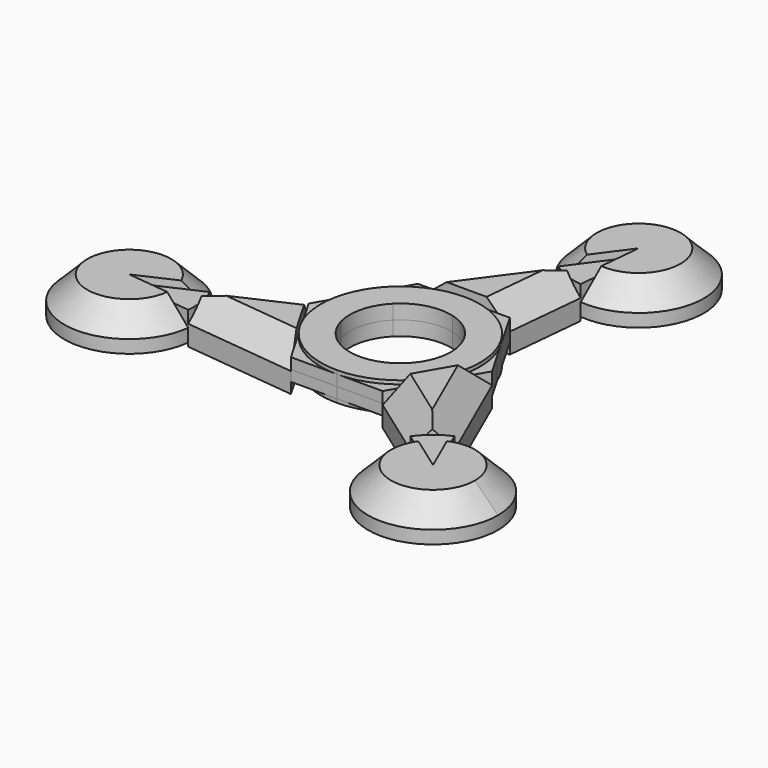
from build123d import *

# Parameters (mm, degrees)
F1_DEPTH      = 3.175
F1_DEPTH_BACK = 3.175
F2_DEPTH      = 2.38125
F2_DEPTH_BACK = 2.38125
F3_DEPTH      = 4.7625
F3_DEPTH_BACK = 4.7625
F4_DEPTH      = 3.96875
F4_DEPTH_BACK = 3.96875
F5_DEPTH      = 2.38125
F5_DEPTH_BACK = 2.38125
F6_T1_DEPTH   = 51.0658567028
F6_T3_DEPTH   = 43.5956947451
F6_2_T1_DEPTH = 43.5956947451
F6_2_T3_DEPTH = 51.0658567028
F6_3_T1_DEPTH = 43.5956947451
F6_3_T3_DEPTH = 51.0658567028
F6_4_T2_ANGLE = 359.64
F6_5_T2_ANGLE = 359.64
F6_6_T2_ANGLE = 268.0514708104
F6_6_T4_ANGLE = 166.1085533485


# Not quite as in the source:
# - a fillet or chamfer that OpenCascade refuses, or shapes differently, is made with other operations: its cross-section is extruded or revolved along the edge and cut away or added
# - a length typed as a fraction of an inch, garbled in the dataset ("3 / 203.2 mm" for 3/8 in), is restored


with BuildPart() as f1:
    # F0 (on Top) → F1 (new body, two sides)
    with BuildSketch(Plane.XY) as f1_sk:
        with BuildLine():
            Line((-4.5196275751, -16.8674797416), (-2.8761266387, -10.7338507446))
            ThreePointArc((-2.8761266387, -10.7338507446), (-7.8577241059, -7.8577241059), (-10.7338507446, -2.8761266387))
            Line((-10.7338507446, -2.8761266387), (-16.8674797416, -4.5196275751))
            ThreePointArc((-16.8674797416, -4.5196275751), (-16.1332463557, -6.6826093913), (-15.1229686637, -8.7312499131))
            ThreePointArc((-15.1229686637, -8.7312499131), (-10.6304964939, -13.8539326743), (-4.5196275751, -16.8674797416))
        make_face()
        with BuildLine():
            ThreePointArc((-7.8577241059, 7.8577241059), (-2.8761266387, 10.7338507446), (2.8761266387, 10.7338507446))
            Line((2.8761266387, 10.7338507446), (4.5196275751, 16.8674797416))
            ThreePointArc((4.5196275751, 16.8674797416), (2.2793136316, 17.3131058917), (0, 17.4625))
            ThreePointArc((0, 17.4625), (-6.6826094377, 16.1332463365), (-12.3478521665, 12.3478521665))
            Line((-12.3478521665, 12.3478521665), (-7.8577241059, 7.8577241059))
        make_face()
        with BuildLine():
            ThreePointArc((-10.7338507446, -2.8761266387), (-10.7338507446, 2.8761266387), (-7.8577241059, 7.8577241059))
            Line((-7.8577241059, 7.8577241059), (-12.3478521665, 12.3478521665))
            ThreePointArc((-12.3478521665, 12.3478521665), (-13.8539326905, 10.6304964728), (-15.12296859, 8.7312500408))
            ThreePointArc((-15.12296859, 8.7312500408), (-17.3131058887, 2.279313655), (-16.8674797416, -4.5196275751))
            Line((-16.8674797416, -4.5196275751), (-10.7338507446, -2.8761266387))
        make_face()
        with BuildLine():
            ThreePointArc((2.8761266387, 10.7338507446), (7.8577241059, 7.8577241059), (10.7338507446, 2.8761266387))
            Line((10.7338507446, 2.8761266387), (16.8674797416, 4.5196275751))
            ThreePointArc((16.8674797416, 4.5196275751), (16.1332463692, 6.6826093587), (15.122968699, 8.731249852))
            ThreePointArc((15.122968699, 8.731249852), (10.6304965218, 13.8539326528), (4.5196275751, 16.8674797416))
            Line((4.5196275751, 16.8674797416), (2.8761266387, 10.7338507446))
        make_face()
        with BuildLine():
            ThreePointArc((10.7338507446, 2.8761266387), (11.017431022, 1.450472311), (11.1125, 0))
            ThreePointArc((11.1125, 0), (10.266611305, -4.2525696422), (7.8577241059, -7.8577241059))
            Line((7.8577241059, -7.8577241059), (12.3478521665, -12.3478521665))
            ThreePointArc((12.3478521665, -12.3478521665), (13.853932765, -10.6304963756), (15.1229687125, -8.7312498287))
            ThreePointArc((15.1229687125, -8.7312498287), (16.8674797672, -4.5196274796), (17.4625, 0))
            ThreePointArc((17.4625, 0), (17.3131058917, 2.2793136316), (16.8674797416, 4.5196275751))
            Line((16.8674797416, 4.5196275751), (10.7338507446, 2.8761266387))
        make_face()
        with BuildLine():
            Line((12.3478521665, -12.3478521665), (7.8577241059, -7.8577241059))
            ThreePointArc((7.8577241059, -7.8577241059), (2.8761266387, -10.7338507446), (-2.8761266387, -10.7338507446))
            Line((-2.8761266387, -10.7338507446), (-4.5196275751, -16.8674797416))
            ThreePointArc((-4.5196275751, -16.8674797416), (-2.2793136142, -17.313105894), (3.53e-08, -17.4625))
            ThreePointArc((3.53e-08, -17.4625), (6.682609454, -16.1332463297), (12.3478521665, -12.3478521665))
        make_face()
    extrude(amount=-F1_DEPTH)
    extrude(f1_sk.sketch, amount=F1_DEPTH_BACK)

    # F0 (on Top) → F2 (join, two sides)
    with BuildSketch(Plane.XY) as f2_sk:
        with BuildLine():
            Line((4.6790627728, 17.4625), (4.5196275751, 16.8674797416))
            ThreePointArc((4.5196275751, 16.8674797416), (10.6304965218, 13.8539326528), (15.122968699, 8.731249852))
            Line((15.122968699, 8.731249852), (10.0819790757, 17.4625))
            Line((10.0819790757, 17.4625), (4.6790627728, 17.4625))
        make_face()
        with BuildLine():
            Line((17.4625, 4.6790627728), (16.8674797416, 4.5196275751))
            ThreePointArc((16.8674797416, 4.5196275751), (17.3131058917, 2.2793136316), (17.4625, 0))
            ThreePointArc((17.4625, 0), (16.8674797672, -4.5196274796), (15.1229687125, -8.7312498287))
            Line((15.1229687125, -8.7312498287), (20.1639581514, 0))
            Line((20.1639581514, 0), (17.4625, 4.6790627728))
        make_face()
        with BuildLine():
            Line((12.7834372272, -12.7834372272), (12.3478521665, -12.3478521665))
            ThreePointArc((12.3478521665, -12.3478521665), (6.682609454, -16.1332463297), (3.53e-08, -17.4625))
            Line((3.53e-08, -17.4625), (10.0819790757, -17.4625))
            Line((10.0819790757, -17.4625), (12.7834372272, -12.7834372272))
        make_face()
        with BuildLine():
            Line((-4.6790627728, -17.4625), (-4.5196275751, -16.8674797416))
            ThreePointArc((-4.5196275751, -16.8674797416), (-10.6304964939, -13.8539326743), (-15.1229686637, -8.7312499131))
            Line((-15.1229686637, -8.7312499131), (-10.0819790757, -17.4625))
            Line((-10.0819790757, -17.4625), (-4.6790627728, -17.4625))
        make_face()
        with BuildLine():
            Line((-17.4625, -4.6790627728), (-16.8674797416, -4.5196275751))
            ThreePointArc((-16.8674797416, -4.5196275751), (-17.3131058887, 2.279313655), (-15.12296859, 8.7312500408))
            Line((-15.12296859, 8.7312500408), (-20.1639581514, 0))
            Line((-20.1639581514, 0), (-17.4625, -4.6790627728))
        make_face()
        with BuildLine():
            Line((-12.7834372272, 12.7834372272), (-12.3478521665, 12.3478521665))
            ThreePointArc((-12.3478521665, 12.3478521665), (-6.6826094377, 16.1332463365), (0, 17.4625))
            Line((0, 17.4625), (-10.0819790757, 17.4625))
            Line((-10.0819790757, 17.4625), (-12.7834372272, 12.7834372272))
        make_face()
        with BuildLine():
            ThreePointArc((-15.12296859, 8.7312500408), (-13.8539326905, 10.6304964728), (-12.3478521665, 12.3478521665))
            Line((-12.3478521665, 12.3478521665), (-12.7834372272, 12.7834372272))
            Line((-12.7834372272, 12.7834372272), (-15.12296859, 8.7312500408))
        make_face()
        with BuildLine():
            ThreePointArc((-15.1229686637, -8.7312499131), (-16.1332463557, -6.6826093913), (-16.8674797416, -4.5196275751))
            Line((-16.8674797416, -4.5196275751), (-17.4625, -4.6790627728))
            Line((-17.4625, -4.6790627728), (-15.1229686637, -8.7312499131))
        make_face()
        with BuildLine():
            ThreePointArc((3.53e-08, -17.4625), (-2.2793136142, -17.313105894), (-4.5196275751, -16.8674797416))
            Line((-4.5196275751, -16.8674797416), (-4.6790627728, -17.4625))
            Line((-4.6790627728, -17.4625), (3.53e-08, -17.4625))
        make_face()
        with BuildLine():
            ThreePointArc((15.1229687125, -8.7312498287), (13.853932765, -10.6304963756), (12.3478521665, -12.3478521665))
            Line((12.3478521665, -12.3478521665), (12.7834372272, -12.7834372272))
            Line((12.7834372272, -12.7834372272), (15.1229687125, -8.7312498287))
        make_face()
        with BuildLine():
            ThreePointArc((15.122968699, 8.731249852), (16.1332463692, 6.6826093587), (16.8674797416, 4.5196275751))
            Line((16.8674797416, 4.5196275751), (17.4625, 4.6790627728))
            Line((17.4625, 4.6790627728), (15.122968699, 8.731249852))
        make_face()
        with BuildLine():
            ThreePointArc((0, 17.4625), (2.2793136316, 17.3131058917), (4.5196275751, 16.8674797416))
            Line((4.5196275751, 16.8674797416), (4.6790627728, 17.4625))
            Line((4.6790627728, 17.4625), (0, 17.4625))
        make_face()
    extrude(amount=F2_DEPTH)
    extrude(f2_sk.sketch, amount=-F2_DEPTH_BACK)


with BuildPart() as f3:
    # F0 (on Top) → F3 (new body, two sides)
    with BuildSketch(Plane.XY) as f3_sk:
        with BuildLine():
            Line((25.8182363481, -25.8182363481), (12.7834372272, -12.7834372272))
            Line((12.7834372272, -12.7834372272), (10.0819790757, -17.4625))
            Line((10.0819790757, -17.4625), (24.2952466492, -27.6159690372))
            ThreePointArc((24.2952466492, -27.6159690372), (25.0196206528, -26.6856549328), (25.8182363481, -25.8182363481))
        make_face()
        with BuildLine():
            Line((20.1639581514, 0), (15.1229687125, -8.7312498287))
            Line((15.1229687125, -8.7312498287), (12.7834372272, -12.7834372272))
            Line((12.7834372272, -12.7834372272), (25.8182363481, -25.8182363481))
            ThreePointArc((25.8182363481, -25.8182363481), (27.8608858867, -24.1241256529), (30.1816043452, -22.8369993881))
            Line((30.1816043452, -22.8369993881), (20.1639581514, 0))
        make_face()
    extrude(amount=F3_DEPTH)
    extrude(f3_sk.sketch, amount=-F3_DEPTH_BACK)

    # F6: chamfer of 5.08 on 2 edges, made by hand

    # F6_s2 → F6_t1 (cut)
    with BuildSketch(Plane(origin=(18.5194987555, -42.2184786293, 0), x_dir=(0, 0, 1), z_dir=(-0.4017091961, 0.9157672858, 0))):
        Polygon((-0.3175, 18.4654932278), (4.7625, 13.3854932278), (4.7625, 18.4654932278), align=None)
    extrude(amount=F6_T1_DEPTH, mode=Mode.SUBTRACT)

    # F6_s4 → F6_t3 (cut)
    with BuildSketch(Plane(origin=(4.3046564772, -3.0750983918, 0), x_dir=(0, 0, 1), z_dir=(0.8137027356, -0.5812812211, 0))):
        Polygon((-0.3175, 8.348818912), (4.7625, 3.268818912), (4.7625, 8.348818912), align=None)
    extrude(amount=F6_T3_DEPTH, mode=Mode.SUBTRACT)


with BuildPart() as f3b:
    # F0 (on Top) → F3, piece 2 (new body, two sides)
    with BuildSketch(Plane.XY) as f3_2_sk:
        with BuildLine():
            Line((9.4501303843, 35.2683667324), (4.6790627728, 17.4625))
            Line((4.6790627728, 17.4625), (10.0819790757, 17.4625))
            Line((10.0819790757, 17.4625), (11.7685074117, 34.848285308))
            ThreePointArc((11.7685074117, 34.848285308), (10.600644762, 35.0104545447), (9.4501303843, 35.2683667324))
        make_face()
        with BuildLine():
            Line((-10.0819790757, 17.4625), (0, 17.4625))
            Line((0, 17.4625), (4.6790627728, 17.4625))
            Line((4.6790627728, 17.4625), (9.4501303843, 35.2683667324))
            ThreePointArc((9.4501303843, 35.2683667324), (6.9616627161, 36.1902977763), (4.6866194437, 37.556535784))
            Line((4.6866194437, 37.556535784), (-10.0819790757, 17.4625))
        make_face()
    extrude(amount=F3_DEPTH)
    extrude(f3_2_sk.sketch, amount=-F3_DEPTH_BACK)

    # F6#2: chamfer of 5.08 on 2 edges, made by hand

    # F6_2_s2 → F6_2_t1 (cut)
    with BuildSketch(Plane(origin=(0.5107850878, 5.2654910597, 0), x_dir=(0, 0, 1), z_dir=(0.0965529364, 0.9953278507, 0))):
        Polygon((4.7625, 3.268818912), (-0.3175, 8.348818912), (4.7625, 8.348818912), align=None)
    extrude(amount=F6_2_T1_DEPTH, mode=Mode.SUBTRACT)

    # F6_2_s4 → F6_2_t3 (cut)
    with BuildSketch(Plane(origin=(27.3025256244, 37.1475957023, 0), x_dir=(0, 0, 1), z_dir=(-0.5922231354, -0.8057740117, 0))):
        Polygon((-0.3175, 18.4654932278), (4.7625, 13.3854932278), (4.7625, 18.4654932278), align=None)
    extrude(amount=F6_2_T3_DEPTH, mode=Mode.SUBTRACT)


with BuildPart() as f3c:
    # F0 (on Top) → F3, piece 3 (new body, two sides)
    with BuildSketch(Plane.XY) as f3_3_sk:
        with BuildLine():
            Line((-10.0819790757, -17.4625), (-15.1229686637, -8.7312499131))
            Line((-15.1229686637, -8.7312499131), (-17.4625, -4.6790627728))
            Line((-17.4625, -4.6790627728), (-35.2683667324, -9.4501303843))
            ThreePointArc((-35.2683667324, -9.4501303843), (-34.9037635186, -11.2831145199), (-34.7815319755, -13.1480074912))
            ThreePointArc((-34.7815319755, -13.1480074912), (-34.8032213919, -13.9349666021), (-34.8682237889, -14.7195363959))
            Line((-34.8682237889, -14.7195363959), (-10.0819790757, -17.4625))
        make_face()
        with BuildLine():
            Line((-35.2683667324, -9.4501303843), (-17.4625, -4.6790627728))
            Line((-17.4625, -4.6790627728), (-20.1639581514, 0))
            Line((-20.1639581514, 0), (-36.0637540609, -7.2323162708))
            ThreePointArc((-36.0637540609, -7.2323162708), (-35.6202654148, -8.324799612), (-35.2683667324, -9.4501303843))
        make_face()
    extrude(amount=F3_DEPTH)
    extrude(f3_3_sk.sketch, amount=-F3_DEPTH_BACK)

    # F6#3: chamfer of 5.08 on 2 edges, made by hand

    # F6_3_s2 → F6_3_t1 (cut)
    with BuildSketch(Plane(origin=(-4.815441565, -2.1903926679, 0), x_dir=(0, 0, 1), z_dir=(-0.9102556721, -0.4140466296, 0))):
        Polygon((-0.3175, 8.348818912), (4.7625, 3.268818912), (4.7625, 8.348818912), align=None)
    extrude(amount=F6_3_T1_DEPTH, mode=Mode.SUBTRACT)

    # F6_3_s4 → F6_3_t3 (cut)
    with BuildSketch(Plane(origin=(-45.8220243799, 5.070882927, 0), x_dir=(0, 0, 1), z_dir=(0.9939323315, -0.1099932742, 0))):
        Polygon((-0.3175, 18.4654932278), (4.7625, 13.3854932278), (4.7625, 18.4654932278), align=None)
    extrude(amount=F6_3_T3_DEPTH, mode=Mode.SUBTRACT)


with BuildPart() as f4:
    # F0 (on Top) → F4 (new body, two sides)
    with BuildSketch(Plane.XY) as f4_sk:
        with BuildLine():
            Line((13.1480074912, 49.0690319755), (11.7685074117, 34.848285308))
            ThreePointArc((11.7685074117, 34.848285308), (22.7506906804, 38.4897535588), (27.4355074912, 49.0690319755))
            ThreePointArc((27.4355074912, 49.0690319755), (6.6966287811, 61.8170659019), (4.6866194437, 37.556535784))
            Line((4.6866194437, 37.556535784), (13.1480074912, 49.0690319755))
        make_face()
    extrude(amount=F4_DEPTH)
    extrude(f4_sk.sketch, amount=-F4_DEPTH_BACK)

    # F6#4: chamfer of 5.08 on 1 edges, made by hand

    # F6_4_s1 → F6_4_t2 (revolve, cut)
    with BuildSketch(Plane(origin=(-5.042448021, 1.9465092507, 0), x_dir=(0, 0, 1), z_dir=(0.9329044068, -0.3601241005, 0))):
        Polygon((3.96875, -41.3041305388), (-1.11125, -36.2241305388), (3.96875, -36.2241305388), align=None)
    revolve(axis=Axis((13.1480074912, 49.0690319755, 3.96875), (0, 0, -1)), revolution_arc=F6_4_T2_ANGLE, mode=Mode.SUBTRACT)


with BuildPart() as f4b:
    # F0 (on Top) → F4, piece 2 (new body, two sides)
    with BuildSketch(Plane.XY) as f4_2_sk:
        with BuildLine():
            ThreePointArc((-36.0637540609, -7.2323162708), (-63.1778021748, -15.4008411988), (-34.8682237889, -14.7195363959))
            Line((-34.8682237889, -14.7195363959), (-49.0690319755, -13.1480074912))
            Line((-49.0690319755, -13.1480074912), (-36.0637540609, -7.2323162708))
        make_face()
    extrude(amount=F4_DEPTH)
    extrude(f4_2_sk.sketch, amount=-F4_DEPTH_BACK)

    # F6#5: chamfer of 5.08 on 1 edges, made by hand

    # F6_5_s1 → F6_5_t2 (revolve, cut)
    with BuildSketch(Plane(origin=(0.8179896941, -5.0214395273, 0), x_dir=(0, 0, 1), z_dir=(0.1607801593, -0.9869902433, 0))):
        Polygon((-1.11125, 36.2570945471), (3.96875, 41.3370945471), (3.96875, 36.2570945471), align=None)
    revolve(axis=Axis((-49.0690319755, -13.1480074912, 3.96875), (0, 0, 1)), revolution_arc=F6_5_T2_ANGLE, mode=Mode.SUBTRACT)


with BuildPart() as f4c:
    # F0 (on Top) → F4, piece 3 (new body, two sides)
    with BuildSketch(Plane.XY) as f4_3_sk:
        with BuildLine():
            ThreePointArc((50.2085244843, -35.9210244843), (43.7354563578, -23.9599496687), (30.1816043452, -22.8369993881))
            Line((30.1816043452, -22.8369993881), (35.9210244843, -35.9210244843))
            Line((35.9210244843, -35.9210244843), (24.2952466492, -27.6159690372))
            ThreePointArc((24.2952466492, -27.6159690372), (31.5604422163, -49.526831279), (50.2085244843, -35.9210244843))
        make_face()
    extrude(amount=F4_DEPTH)
    extrude(f4_3_sk.sketch, amount=-F4_DEPTH_BACK)

    # F6#6: chamfer of 5.08 on 2 edges, made by hand

    # F6_6_s1 → F6_6_t2 (revolve, cut)
    with BuildSketch(Plane(origin=(34.6588261556, 1.1791406399, 0), x_dir=(0, 0, 1), z_dir=(0.9994217752, 0.0340016949, 0))):
        Polygon((-1.11125, 22.8341297711), (3.96875, 27.9141297711), (3.96875, 22.8341297711), align=None)
    revolve(axis=Axis((35.9210244843, -35.9210244843, 3.96875), (0, 0, 1)), revolution_arc=F6_6_T2_ANGLE, mode=Mode.SUBTRACT)

    # F6_6_s3 → F6_6_t4 (revolve, cut)
    with BuildSketch(Plane.XZ.offset(35.9210244843)):
        Polygon((45.1285244843, 3.96875), (50.2085244843, -1.11125), (50.2085244843, 3.96875), align=None)
    revolve(axis=Axis((35.9210244843, -35.9210244843, 3.96875), (0, 0, 1)), revolution_arc=F6_6_T4_ANGLE, mode=Mode.SUBTRACT)


with BuildPart() as f5:
    # F0 (on Top) → F5 (new body, two sides)
    with BuildSketch(Plane.XY) as f5_sk:
        with BuildLine():
            Line((35.9210244843, -35.9210244843), (25.8182363481, -25.8182363481))
            ThreePointArc((25.8182363481, -25.8182363481), (25.0196206528, -26.6856549328), (24.2952466492, -27.6159690372))
            Line((24.2952466492, -27.6159690372), (35.9210244843, -35.9210244843))
        make_face()
        with BuildLine():
            ThreePointArc((30.1816043452, -22.8369993881), (27.8608858867, -24.1241256529), (25.8182363481, -25.8182363481))
            Line((25.8182363481, -25.8182363481), (35.9210244843, -35.9210244843))
            Line((35.9210244843, -35.9210244843), (30.1816043452, -22.8369993881))
        make_face()
    extrude(amount=F5_DEPTH)
    extrude(f5_sk.sketch, amount=-F5_DEPTH_BACK)


with BuildPart() as f5b:
    # F0 (on Top) → F5, piece 2 (new body, two sides)
    with BuildSketch(Plane.XY) as f5_2_sk:
        with BuildLine():
            Line((13.1480074912, 49.0690319755), (9.4501303843, 35.2683667324))
            ThreePointArc((9.4501303843, 35.2683667324), (10.600644762, 35.0104545447), (11.7685074117, 34.848285308))
            Line((11.7685074117, 34.848285308), (13.1480074912, 49.0690319755))
        make_face()
        with BuildLine():
            ThreePointArc((4.6866194437, 37.556535784), (6.9616627161, 36.1902977763), (9.4501303843, 35.2683667324))
            Line((9.4501303843, 35.2683667324), (13.1480074912, 49.0690319755))
            Line((13.1480074912, 49.0690319755), (4.6866194437, 37.556535784))
        make_face()
    extrude(amount=F5_DEPTH)
    extrude(f5_2_sk.sketch, amount=-F5_DEPTH_BACK)


with BuildPart() as f5c:
    # F0 (on Top) → F5, piece 3 (new body, two sides)
    with BuildSketch(Plane.XY) as f5_3_sk:
        with BuildLine():
            Line((-49.0690319755, -13.1480074912), (-35.2683667324, -9.4501303843))
            ThreePointArc((-35.2683667324, -9.4501303843), (-35.6202654148, -8.324799612), (-36.0637540609, -7.2323162708))
            Line((-36.0637540609, -7.2323162708), (-49.0690319755, -13.1480074912))
        make_face()
        with BuildLine():
            ThreePointArc((-34.7815319755, -13.1480074912), (-34.9037635186, -11.2831145199), (-35.2683667324, -9.4501303843))
            Line((-35.2683667324, -9.4501303843), (-49.0690319755, -13.1480074912))
            Line((-49.0690319755, -13.1480074912), (-34.8682237889, -14.7195363959))
            ThreePointArc((-34.8682237889, -14.7195363959), (-34.8032213919, -13.9349666021), (-34.7815319755, -13.1480074912))
        make_face()
    extrude(amount=F5_DEPTH)
    extrude(f5_3_sk.sketch, amount=-F5_DEPTH_BACK)


solid = Compound([f1.part, f3.part, f3b.part, f3c.part, f4.part, f4b.part, f4c.part, f5.part, f5b.part, f5c.part])
